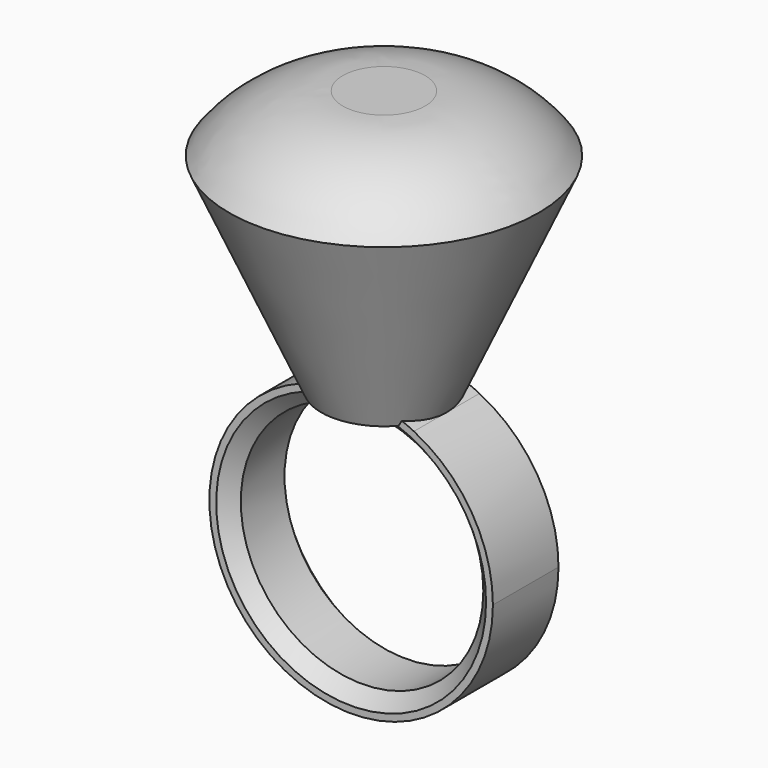
from build123d import *

# Parameters (mm, degrees)
F0_R          = 8.875
F3_DEPTH      = 3
F3_DEPTH_BACK = 3


# Not quite as in the source:
# - a fillet or chamfer that OpenCascade refuses, or shapes differently, is made with other operations: its cross-section is extruded or revolved along the edge and cut away or added


with BuildPart() as f2:
    # F0 (on Front) → F2 (revolve)
    with BuildSketch(Plane.XZ):
        with BuildLine():
            ThreePointArc((0, 10.375), (2.35804, 10.103478), (4.592657, 9.303125))
            Line((4.592657, 9.303125), (11.330436, 24.349924))
            ThreePointArc((11.330436, 24.349924), (7.667321, 27.423958), (3.01418, 28.526856))
            Line((3.01418, 28.526856), (0, 28.526856))
            Line((0, 28.526856), (0, 10.375))
        make_face()
        with BuildLine():
            Line((0, 9.303125), (4.592657, 9.303125))
            ThreePointArc((4.592657, 9.303125), (2.35804, 10.103478), (0, 10.375))
            Line((0, 10.375), (0, 9.303125))
        make_face()
    revolve(axis=Axis((0, 0, 0), (0, 0, 1)))

    # F0 (on Front) → F3 (join, two sides)
    with BuildSketch(Plane.XZ) as f3_sk:
        with BuildLine():
            ThreePointArc((0, 10.375), (-7.336233, -7.336233), (10.375, 0))
            ThreePointArc((10.375, 0), (8.811624, 5.476852), (4.592657, 9.303125))
            Line((4.592657, 9.303125), (0, 9.303125))
            Line((0, 9.303125), (0, 10.375))
        make_face()
        Circle(F0_R, mode=Mode.SUBTRACT)
        with BuildLine():
            Line((0, 9.303125), (4.592657, 9.303125))
            ThreePointArc((4.592657, 9.303125), (2.35804, 10.103478), (0, 10.375))
            Line((0, 10.375), (0, 9.303125))
        make_face()
    extrude(amount=F3_DEPTH)
    extrude(f3_sk.sketch, amount=-F3_DEPTH_BACK)

    # F4: chamfer of 1 on 2 edges, made by hand


with BuildPart() as f4_tool2:
    # F4_s3 → F4_t4 (revolve)
    with BuildSketch(Plane.XY):
        Polygon((9.875, -3), (8.875, -2), (8.875, -3), align=None)
    revolve(axis=Axis((0, -3, 0), (0, -1, 0)))

    split(bisect_by=Plane.XY.offset(9.303125), keep=Keep.BOTTOM)


with BuildPart() as f2_1:
    add(f2.part)

    # F4_t1: cut F4_tool2
    add(f4_tool2.part, mode=Mode.SUBTRACT)


with BuildPart() as f4_tool7:
    # F4_s8 → F4_t9 (revolve)
    with BuildSketch(Plane.XY):
        Polygon((8.875, 2), (9.875, 3), (8.875, 3), align=None)
    revolve(axis=Axis((0, 3, 0), (0, -1, 0)))

    split(bisect_by=Plane.XY.offset(9.303125), keep=Keep.BOTTOM)


with BuildPart() as f2_2:
    add(f2_1.part)

    # F4_t6: cut F4_tool7
    add(f4_tool7.part, mode=Mode.SUBTRACT)


solid = f2_2.part
